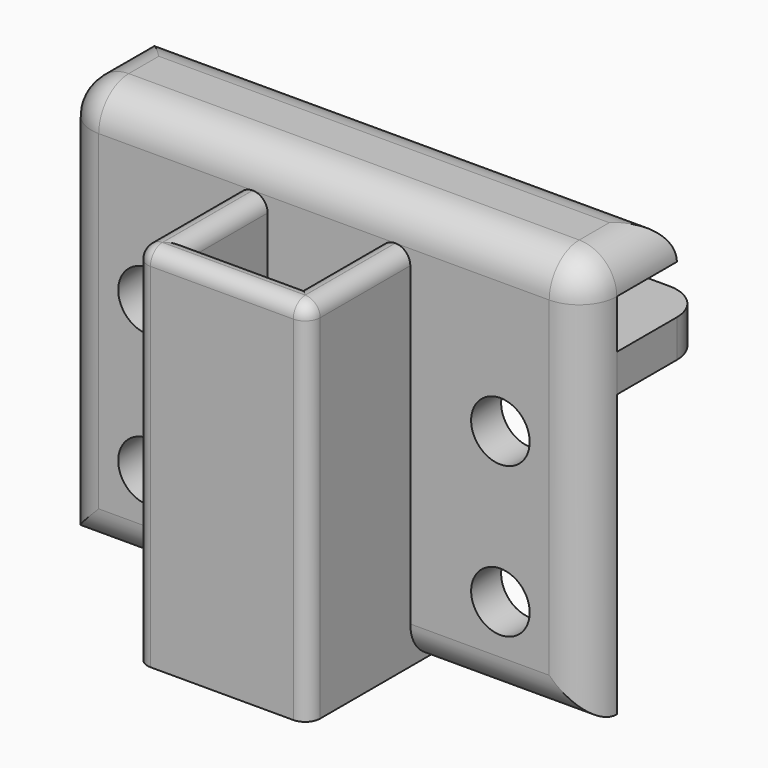
from build123d import *

# Parameters (mm, degrees)
F1_DEPTH       = 35
F1_DEPTH_BACK  = 35
F3_DEPTH       = 49
F4_R           = 1.99
F5_R           = 3.9
F6_DEPTH       = 25
F8_DEPTH       = 2.5
F10_DEPTH      = 11.5
F10_DEPTH_BACK = 11.5
F11_R          = 4.99999


# Not quite as in the source:
# - a fillet or chamfer is up to 0.001 mm smaller than in the source, because OpenCascade refuses the exact size


with BuildPart() as f1:
    # F0 (on Right) → F1 (new body, two sides)
    with BuildSketch(Plane.YZ) as f1_sk:
        Polygon((15, 0), (0, 0), (0, 6.5), (10, 6.5), (10, 11.5), (-5, 11.5), (-5, -5), (-5, -42.5), (0, -42.5), (0, -5), (15, -5), align=None)
    extrude(amount=F1_DEPTH)
    extrude(f1_sk.sketch, amount=-F1_DEPTH_BACK)

    # F2 (on face) → F3 (join, through all)
    with BuildSketch(Plane(origin=(0, 0, 6.5), x_dir=(1, 0, 0), z_dir=(0, 0, -1))):
        Polygon((7.5, 18), (7.5, 5), (11.5, 5), (11.5, 22), (0, 22), (-11.5, 22), (-11.5, 5), (-7.5, 5), (-7.5, 18), (0, 18), align=None)
    extrude(amount=F3_DEPTH)

    # F4
    f4_edges = [f1.edges().sort_by_distance(p)[0] for p in [
        (11.5, -13.5, 6.5),
        (7.5, -11.5, 6.5),
        (-7.5, -11.5, 6.5),
        (0, -18, 6.5),
        (0, -22, 6.5),
        (-11.5, -13.5, 6.5),
        (-11.5, -22, -18),
        (11.5, -22, -18),
    ]]
    fillet(f4_edges, radius=F4_R)

    # F5 (on face) → F6 (cut)
    with BuildSketch(Plane.XZ.offset(5)):
        with Locations((23.5, -11)):
            Circle(F5_R)
        with Locations((23.5, -31)):
            Circle(F5_R)
        with Locations((-23.5, -11)):
            Circle(F5_R)
        with Locations((-23.5, -31)):
            Circle(F5_R)
    extrude(amount=-F6_DEPTH, mode=Mode.SUBTRACT)

    # F7 (on face) → F8 (join)
    with BuildSketch(Plane(origin=(0, 0, -42.5), x_dir=(1, 0, 0), z_dir=(0, 0, -1))):
        Polygon((1.5, 18), (0, 18), (-1.5, 18), (-1.5, 13), (-7.5, 13), (-7.5, 11.5), (-7.5, 10), (-1.5, 10), (-1.5, 5), (0, 5), (1.5, 5), (1.5, 10), (7.5, 10), (7.5, 11.5), (7.5, 13), (1.5, 13), align=None)
    extrude(amount=-F8_DEPTH)

    # F9 (on Right) → F10 (join, two sides)
    with BuildSketch(Plane.YZ) as f10_sk:
        Polygon((0, -5), (0, -42.5), (15, -5), align=None)
    extrude(amount=-F10_DEPTH)
    extrude(f10_sk.sketch, amount=F10_DEPTH_BACK)

    # F11 (radius 5 in the source; OpenCascade refuses exactly that, so slightly less here)
    f11_edges = [f1.edges().sort_by_distance(p)[0] for p in [
        (-23.25, -5, -42.5),
        (23.25, -5, -42.5),
        (0, 10, 11.5),
        (35, 2.5, 11.5),
        (-35, 2.5, 11.5),
        (0, -5, 11.5),
        (-35, -5, -15.5),
        (35, -5, -15.5),
        (11.5, 7.5, -23.75),
        (-11.5, 7.5, -23.75),
        (35, 15, -2.5),
        (-35, 15, -2.5),
    ]]
    fillet(f11_edges, radius=F11_R)


solid = f1.part
